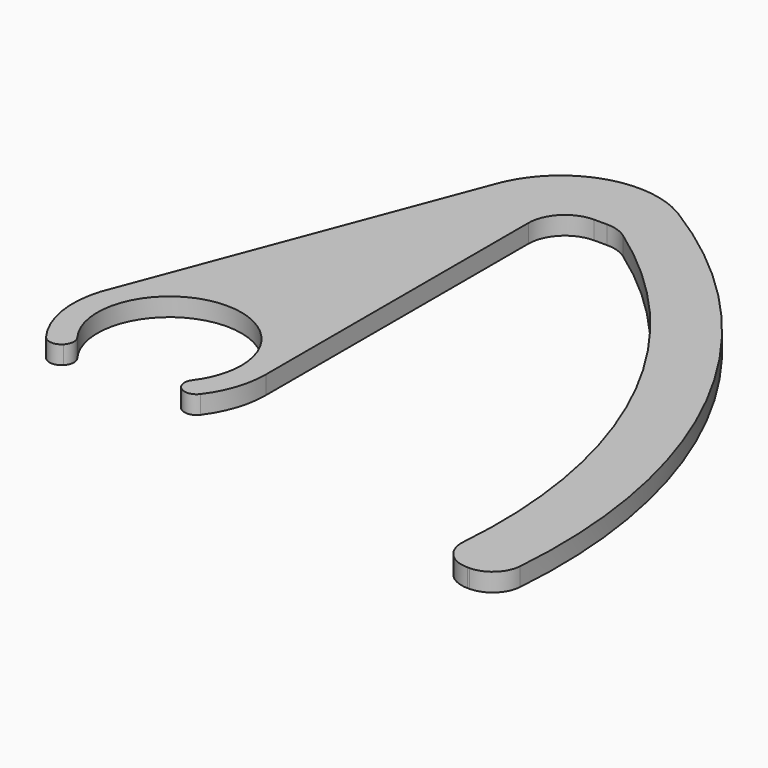
from build123d import *

# Parameters (mm, degrees)
F1_DEPTH = 1.5
F2_R     = 3
F3_R     = 2.4
F4_R     = 0.99999
F5_R     = 8


# Not quite as in the source:
# - a fillet or chamfer is up to 0.001 mm smaller than in the source, because OpenCascade refuses the exact size


with BuildPart() as f1:
    # F0 (on Top) → F1 (new body)
    with BuildSketch(Plane.XY):
        with BuildLine():
            ThreePointArc((-7.2162480919, 3.2149282225), (1.6434171829, 7.7271715371), (7.9, 0))
            Line((7.9, 0), (7.9, 29.9))
            Line((7.9, 29.9), (2.9, 29.9))
            Line((2.9, 29.9), (-7.2162480919, 3.2149282225))
        make_face()
        with BuildLine():
            Line((2.9, 29.9), (7.9, 29.9))
            Line((7.9, 29.9), (12.9, 29.9))
            ThreePointArc((12.9, 29.9), (28.5747012766, 11.2865794971), (31.9942384958, -12.8062088042))
            Line((31.9942384958, -12.8062088042), (36.9942384958, -12.8062088042))
            ThreePointArc((36.9942384958, -12.8062088042), (32.2218442931, 14.721028685), (12.9, 34.9))
            ThreePointArc((12.9, 34.9), (6.9234468079, 34.3531063842), (2.9, 29.9))
        make_face()
        with BuildLine():
            ThreePointArc((5.9, 0), (5.4508892418, -2.257832251), (4.171930009, -4.171930009))
            Line((4.171930009, -4.171930009), (5.5861435714, -5.5861435714))
            ThreePointArc((5.5861435714, -5.5861435714), (7.2986483068, -3.0231991157), (7.9, 0))
            ThreePointArc((7.9, 0), (1.6434171829, 7.7271715371), (-7.2162480919, 3.2149282225))
            ThreePointArc((-7.2162480919, 3.2149282225), (-7.7678841556, -1.4387410276), (-5.5861435714, -5.5861435714))
            Line((-5.5861435714, -5.5861435714), (-4.171930009, -4.171930009))
            ThreePointArc((-4.171930009, -4.171930009), (-2.257832251, 5.4508892418), (5.9, 0))
        make_face()
    extrude(amount=F1_DEPTH)

    # F2
    f2_edges = [f1.edges().sort_by_distance(p)[0] for p in [
        (7.9, 29.9, 0.75),
        (12.9, 29.9, 0.75),
    ]]
    fillet(f2_edges, radius=F2_R)

    # F3
    f3_edges = [f1.edges().sort_by_distance(p)[0] for p in [
        (31.994238, -12.806209, 0.75),
        (36.994238, -12.806209, 0.75),
    ]]
    fillet(f3_edges, radius=F3_R)

    # F4 (radius 1 in the source; OpenCascade refuses exactly that, so slightly less here)
    f4_edges = [f1.edges().sort_by_distance(p)[0] for p in [
        (4.17193, -4.17193, 0.75),
        (-4.17193, -4.17193, 0.75),
        (5.586144, -5.586144, 0.75),
        (-5.586144, -5.586144, 0.75),
    ]]
    fillet(f4_edges, radius=F4_R)

    # F5
    f5_edges = [f1.edges().sort_by_distance(p)[0] for p in [
        (12.9, 34.9, 0.75),
    ]]
    fillet(f5_edges, radius=F5_R)


solid = f1.part
